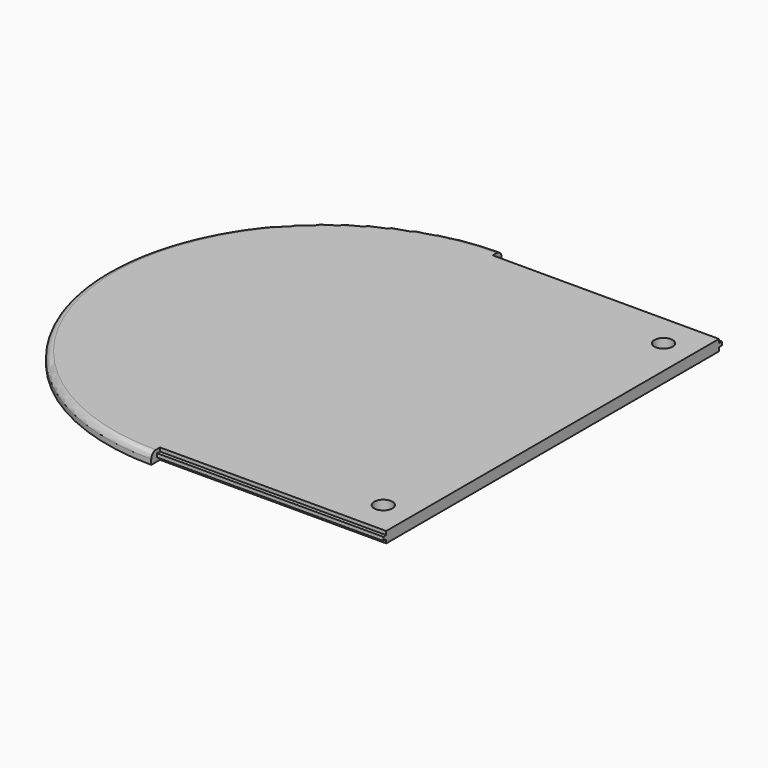
from build123d import *

# Parameters (mm, degrees)
F1_DEPTH = 3.81
F2_W     = 2.54
F2_H     = 3.81
F3_DEPTH = 78.74
F4_W     = 1.27
F4_H     = 1.27
F5_DEPTH = 78.74
F6_R     = 3.175
F7_DEPTH = 25.4
F8_R     = 2.032


# Not quite as in the source:
# - a feature names something its author has since deleted; it is built from what else it names


with BuildPart() as f1:
    # F0 (on Top) → F1 (new body)
    with BuildSketch(Plane.XY):
        with BuildLine():
            Line((0, -76.2), (0, 76.2))
            ThreePointArc((0, 76.2), (-76.2, 0), (0, -76.2))
        make_face()
        with BuildLine():
            ThreePointArc((0, -76.2), (53.8815367264, -53.8815367264), (76.2, 0))
            ThreePointArc((76.2, 0), (53.8815367264, 53.8815367264), (0, 76.2))
            Line((0, 76.2), (0, -76.2))
        make_face()
        with BuildLine():
            ThreePointArc((0, 76.2), (53.8815367264, 53.8815367264), (76.2, 0))
            ThreePointArc((76.2, 0), (53.8815367264, -53.8815367264), (0, -76.2))
            Line((0, -76.2), (78.74, -76.2))
            Line((78.74, -76.2), (78.74, 76.2))
            Line((78.74, 76.2), (0, 76.2))
        make_face()
    extrude(amount=F1_DEPTH)

    # F2 (on face) → F3 (cut)
    with BuildSketch(Plane.YZ.offset(78.74)):
        with Locations((-74.93, 1.905)):
            Rectangle(F2_W, F2_H)
        with Locations((74.93, 1.905)):
            Rectangle(F2_W, F2_H)
    extrude(amount=-F3_DEPTH, mode=Mode.SUBTRACT)

    # F4 (on face) → F5 (cut)
    with BuildSketch(Plane.YZ.offset(78.74)):
        with Locations((-73.025, 3.175)):
            Rectangle(F4_W, F4_H)
        with Locations((-73.025, 0.635)):
            Rectangle(F4_W, F4_H)
        with Locations((73.025, 3.175)):
            Rectangle(F4_W, F4_H)
        with Locations((73.025, 0.635)):
            Rectangle(F4_W, F4_H)
    extrude(amount=-F5_DEPTH, mode=Mode.SUBTRACT)

    # F6 (on face) → F7 (cut)
    with BuildSketch(Plane.XY.offset(3.81)):
        with Locations((68.58, 60.96)):
            Circle(F6_R)
        with Locations((68.58, -60.96)):
            Circle(F6_R)
    extrude(amount=-F7_DEPTH, mode=Mode.SUBTRACT)

    # F8
    f8_edges = [f1.edges().sort_by_distance(p)[0] for p in [
        (-76.2, 0, 3.81),
    ]]
    fillet(f8_edges, radius=F8_R)


solid = f1.part
